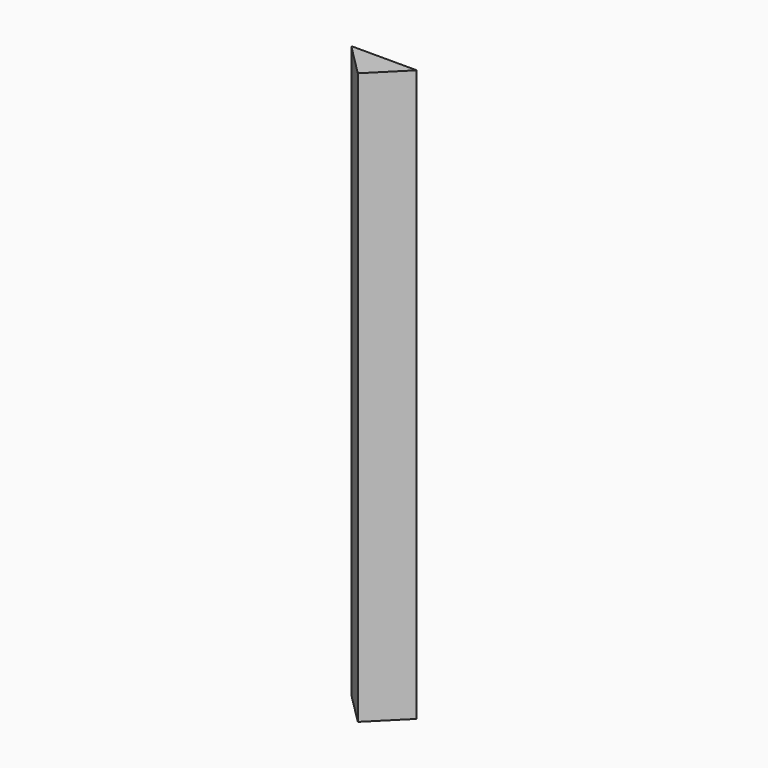
from build123d import *

# Parameters (mm, degrees)
F0_W     = 36
F0_H     = 314
F1_DEPTH = 18
F2_SIZE  = 17.99999


# Not quite as in the source:
# - a fillet or chamfer is up to 0.001 mm smaller than in the source, because OpenCascade refuses the exact size


with BuildPart() as f1:
    # F0 (on Front) → F1 (new body)
    with BuildSketch(Plane.XZ):
        Rectangle(F0_W, F0_H)
    extrude(amount=F1_DEPTH)

    # F2 (size 18 in the source; OpenCascade refuses exactly that, so slightly less here)
    f2_edges = [f1.edges().sort_by_distance(p)[0] for p in [
        (-18, -18, 0),
        (18, -18, 0),
    ]]
    chamfer(f2_edges, length=F2_SIZE)


solid = f1.part
